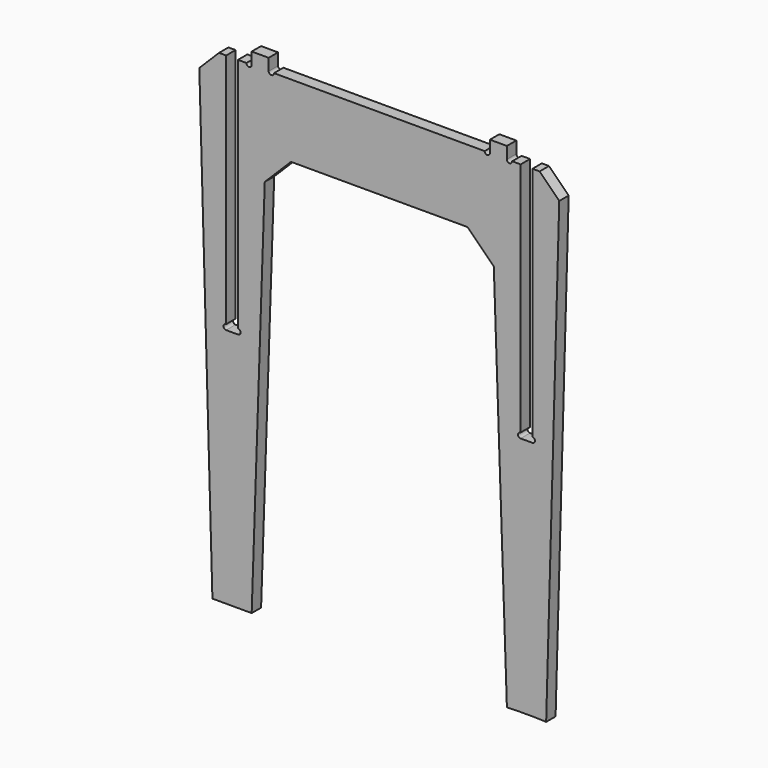
from build123d import *

# Parameters (mm, degrees)
F1_DEPTH = 18


# Not quite as in the source:
# - ends of sketch curves that miss each other by under 0.0002 mm in the source are joined


with BuildPart() as f1:
    # F0 (on Front) → F1 (new body)
    with BuildSketch(Plane.XZ):
        with BuildLine():
            Line((195.0137715405, 361), (195.0137715405, 379))
            Line((195.0137715405, 379), (169.0137715405, 379))
            Line((169.0137715405, 379), (169.0137715405, 361.0021361967))
            Line((169.0137715405, 361.0021361967), (169.0137715405, 361))
            ThreePointArc((169.0137715405, 361), (165.0116353441, 357.0021367671), (161.0137721109, 361.0042723931))
            Line((161.0137721109, 361.0042723931), (-161.0000017113, 361.1762435819))
            ThreePointArc((-161.0000017113, 361.1762435819), (-165.0021373372, 357.1783803487), (-169.0000005704, 361.1805159746))
            Line((-169.0000005704, 361.1805159746), (-169.0000005704, 379.1805159746))
            Line((-169.0000005704, 379.1805159746), (-195.0000005704, 379.1805159746))
            Line((-195.0000005704, 379.1805159746), (-195.0000005704, 361.1805160001))
            ThreePointArc((-195.0000005704, 361.1805160001), (-199, 357.1805165706), (-202.9999994296, 361.1805160001))
            Line((-202.9999994296, 361.1805160001), (-215.9862284595, 361.1805160001))
            Line((-215.9862284595, 361.1805160001), (-215.9862284595, -0.2833213137))
            ThreePointArc((-215.9862284595, -0.2833213137), (-211.9862284595, -4.2833213137), (-215.9862284595, -8.2833213137))
            Line((-215.9862284595, -8.2833213137), (-233.9862284595, -8.2833213137))
            ThreePointArc((-233.9862284595, -8.2833213137), (-237.9862284595, -4.2833213137), (-233.9862284595, -0.2833213137))
            Line((-233.9862284595, -0.2833213137), (-233.9862284595, 361.1805160001))
            Line((-233.9862284595, 361.1805160001), (-244.90749278, 361.1805160001))
            Line((-244.90749278, 361.1805160001), (-274.9862284595, 331.0746893941))
            Line((-274.9862284595, 331.0746893941), (-254.9862284595, -376.2833213137))
            Line((-254.9862284595, -376.2833213137), (-233.9862284595, -376.2833213137))
            Line((-233.9862284595, -376.2833213137), (-215.9862284595, -376.2833213137))
            Line((-215.9862284595, -376.2833213137), (-194.9862284595, -376.2833213137))
            Line((-194.9862284595, -376.2833213137), (-174.9862284595, 210.3365797868))
            Line((-174.9862284595, 210.3365797868), (-134.9862284595, 250.3365797868))
            Line((-134.9862284595, 250.3365797868), (135, 250.3365797868))
            Line((135, 250.3365797868), (175, 210.3365797868))
            Line((175, 210.3365797868), (195, -376.2833213137))
            Line((195, -376.2833213137), (216.0083907756, -375.6897371419))
            Line((216.0083907756, -375.6897371419), (234.0083907756, -375.6897371419))
            Line((234.0083907756, -375.6897371419), (255, -376.2833213137))
            Line((255, -376.2833213137), (275, 331))
            Line((275, 331), (245, 361))
            Line((245, 361), (234.0083907756, 361))
            Line((234.0083907756, 361), (234.0083907756, 0.3102628581))
            ThreePointArc((234.0083907756, 0.3102628581), (238.0083907756, -3.6897371419), (234.0083907756, -7.6897371419))
            Line((234.0083907756, -7.6897371419), (216.0083907756, -7.6897371419))
            ThreePointArc((216.0083907756, -7.6897371419), (212.0083907756, -3.6897371419), (216.0083907756, 0.3102628581))
            Line((216.0083907756, 0.3102628581), (216.0083907756, 361))
            Line((216.0083907756, 361), (203.0137715405, 361))
            ThreePointArc((203.0137715405, 361), (199.0137715405, 357), (195.0137715405, 361))
        make_face()
    extrude(amount=F1_DEPTH)


solid = f1.part
